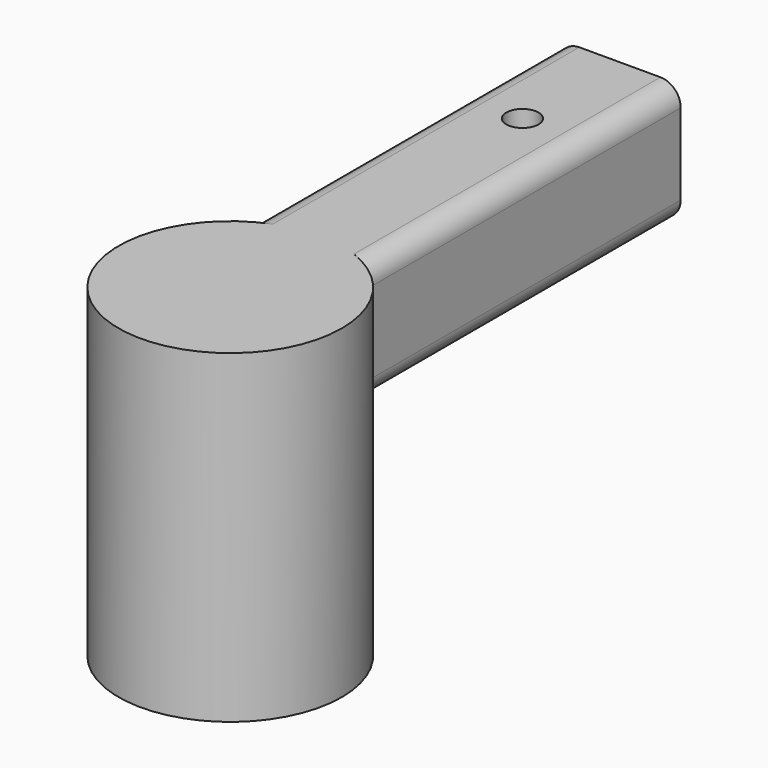
from build123d import *

# Parameters (mm, degrees)
F1_DEPTH = 152.4
F2_R     = 34.925
F3_DEPTH = 101.6
F5_D     = 10.0838


with BuildPart() as f1:
    # F0 (on Front) → F1 (new body)
    with BuildSketch(Plane.XZ):
        with BuildLine():
            ThreePointArc((0, 6.35), (1.8598719395, 1.8598719395), (6.35, 0))
            Line((6.35, 0), (31.75, 0))
            ThreePointArc((31.75, 0), (36.2401280605, 1.8598719395), (38.1, 6.35))
            Line((38.1, 6.35), (38.1, 31.75))
            ThreePointArc((38.1, 31.75), (36.2401280605, 36.2401280605), (31.75, 38.1))
            Line((31.75, 38.1), (6.35, 38.1))
            ThreePointArc((6.35, 38.1), (1.8598719395, 36.2401280605), (0, 31.75))
            Line((0, 31.75), (0, 6.35))
        make_face()
        with BuildLine():
            Line((25.4, 6.35), (12.7, 6.35))
            ThreePointArc((12.7, 6.35), (8.2098719395, 8.2098719395), (6.35, 12.7))
            Line((6.35, 12.7), (6.35, 25.4))
            ThreePointArc((6.35, 25.4), (8.2098719395, 29.8901280605), (12.7, 31.75))
            Line((12.7, 31.75), (25.4, 31.75))
            ThreePointArc((25.4, 31.75), (29.8901280605, 29.8901280605), (31.75, 25.4))
            Line((31.75, 25.4), (31.75, 12.7))
            ThreePointArc((31.75, 12.7), (29.8901280605, 8.2098719395), (25.4, 6.35))
        make_face(mode=Mode.SUBTRACT)
    extrude(amount=F1_DEPTH)

    # F2 (on face) → F3 (join)
    with BuildSketch(Plane.XY.offset(38.1)):
        with Locations((19.05, -152.4)):
            Circle(F2_R)
    extrude(amount=-F3_DEPTH)

    # F5 (through all)
    with Locations(Plane.XY.offset(38.1)):
        with Locations((19.05, -38.1)):
            Hole(F5_D / 2)


solid = f1.part
